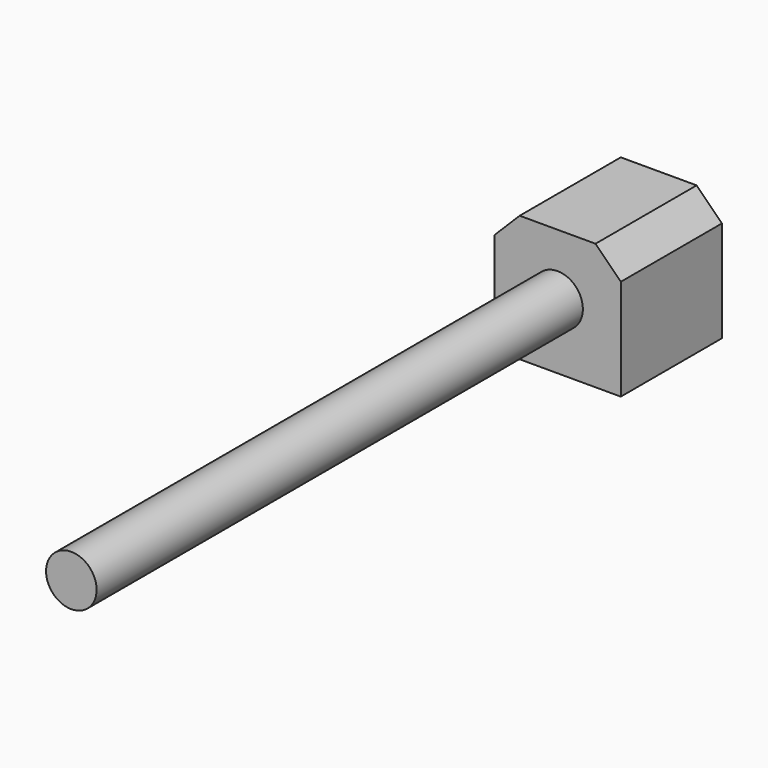
from build123d import *

# Parameters (mm, degrees)
F0_W     = 127
F0_H     = 127
F1_DEPTH = 127
F2_SIZE  = 25.4
F3_R     = 25.4
F4_DEPTH = 610.6993397


# Not quite as in the source:
# - an extrude ends at something that could not be found from the text; its depth is read off the source's solid
# - a feature of the source that left no trace in its solid (it failed there, or was rolled back) is left out


with BuildPart() as f1:
    # F0 (on Front) → F1 (new body)
    with BuildSketch(Plane.XZ):
        with Locations((0, -1.5167773236)):
            Rectangle(F0_W, F0_H)
    extrude(amount=F1_DEPTH)

    # F2
    f2_edges = [f1.edges().sort_by_distance(p)[0] for p in [
        (-63.5, -63.5, 61.983223),
        (63.5, -63.5, 61.983223),
    ]]
    chamfer(f2_edges, length=F2_SIZE)

    # F3 (on face) → F4 (join, through all)
    with BuildSketch(Plane.XZ.offset(127)):
        Circle(F3_R)
    extrude(amount=F4_DEPTH)


solid = f1.part
